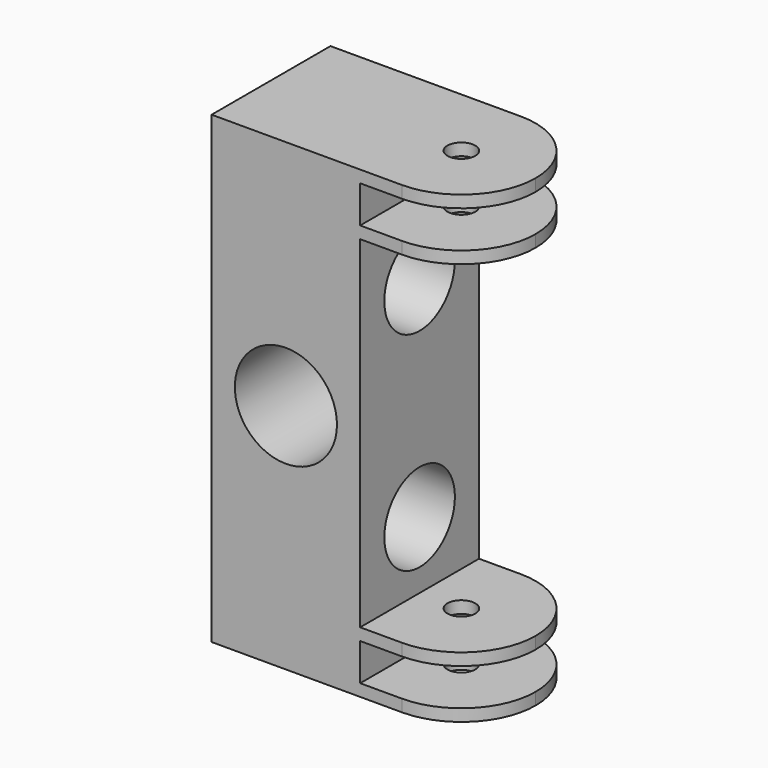
from build123d import *

# Parameters (mm, degrees)
F0_W     = 32
F0_H     = 100
F0_R     = 9.5
F1_DEPTH = 32
F2_R     = 11
F3_DEPTH = 32.001
F4_W     = 32
F4_H     = 2.6
F5_DEPTH = 25
F6_R     = 15.99999
F7_R     = 3
F8_DEPTH = 100.001


# Not quite as in the source:
# - a fillet or chamfer is up to 0.001 mm smaller than in the source, because OpenCascade refuses the exact size


with BuildPart() as f1:
    # F0 (on Right) → F1 (new body)
    with BuildSketch(Plane.YZ):
        Rectangle(F0_W, F0_H)
        with Locations((0, -22.4)):
            Circle(F0_R, mode=Mode.SUBTRACT)
        with Locations((0, 22.4)):
            Circle(F0_R, mode=Mode.SUBTRACT)
    extrude(amount=F1_DEPTH)

    # F2 (on face) → F3 (cut, through all)
    with BuildSketch(Plane.XZ.offset(16)):
        with Locations((16, 0)):
            Circle(F2_R)
    extrude(amount=-F3_DEPTH, mode=Mode.SUBTRACT)

    # F4 (on face) → F5 (join)
    with BuildSketch(Plane.YZ.offset(32)):
        with Locations((0, 48.7)):
            Rectangle(F4_W, F4_H)
        with Locations((0, 38.1)):
            Rectangle(F4_W, F4_H)
        with Locations((0, -38.1)):
            Rectangle(F4_W, F4_H)
        with Locations((0, -48.7)):
            Rectangle(F4_W, F4_H)
    extrude(amount=F5_DEPTH)

    # F6 (radius 16 in the source; OpenCascade refuses exactly that, so slightly less here)
    f6_edges = [f1.edges().sort_by_distance(p)[0] for p in [
        (57, -16, 48.7),
        (57, -16, 38.1),
        (57, 16, 38.1),
        (57, 16, 48.7),
        (57, 16, -48.7),
        (57, -16, -48.7),
        (57, -16, -38.1),
        (57, 16, -38.1),
    ]]
    fillet(f6_edges, radius=F6_R)

    # F7 (on face) → F8 (cut, through all)
    with BuildSketch(Plane.XY.offset(50)):
        with Locations((41, 0)):
            Circle(F7_R)
    extrude(amount=-F8_DEPTH, mode=Mode.SUBTRACT)


solid = f1.part
